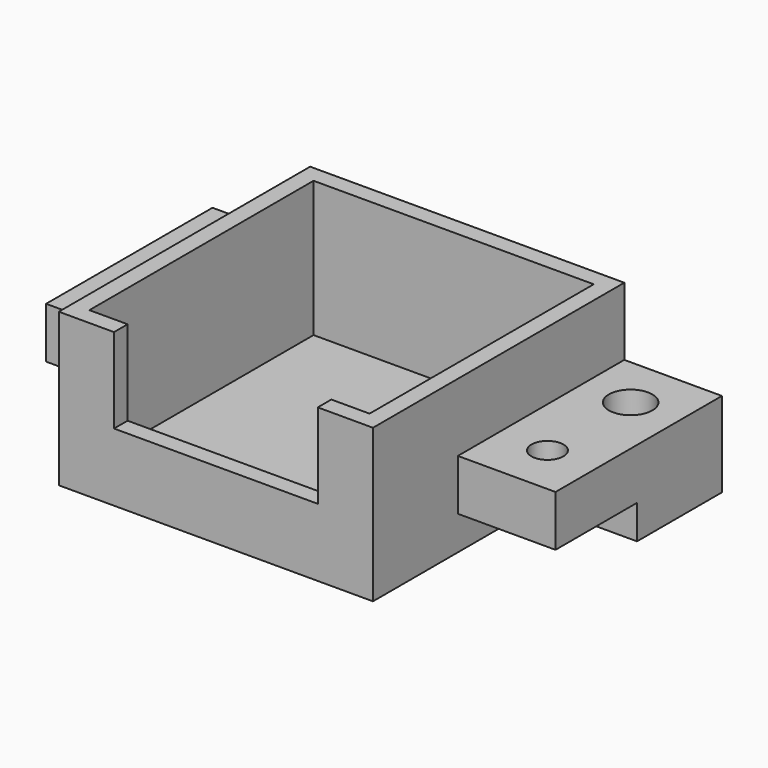
from build123d import *

# Parameters (mm, degrees)
F0_W      = 29.36875
F0_H      = 29.36875
F0_W_2    = 26.19375
F0_H_2    = 26.19375
F1_DEPTH  = 14.2875
F2_W      = 26.19375
F2_H      = 26.19375
F3_DEPTH  = 1.5875
F7_W      = 19.05
F7_H      = 7.9375
F8_DEPTH  = 1.5875
F9_R      = 1.5
F10_DEPTH = 4.7625
F11_R     = 2.032
F12_DEPTH = 7.9375


with BuildPart() as f1:
    # F0 (on Top) → F1 (new body)
    with BuildSketch(Plane.XY):
        Rectangle(F0_W, F0_H)
        Rectangle(F0_W_2, F0_H_2, mode=Mode.SUBTRACT)
    extrude(amount=F1_DEPTH)

    # F2 (on face) → F3 (join)
    with BuildSketch(Plane(origin=(0, 0, 0), x_dir=(1, 0, 0), z_dir=(0, 0, -1))):
        Rectangle(F2_W, F2_H)
    extrude(amount=-F3_DEPTH)

    # F4: union 

    # F7 (on face) → F8 (cut, through all)
    with BuildSketch(Plane.XZ.offset(14.684375)):
        with Locations((0, 10.31875)):
            Rectangle(F7_W, F7_H)
    extrude(amount=-F8_DEPTH, mode=Mode.SUBTRACT)

    # F9 (on face) → F10 (join)
    with BuildSketch(Plane(origin=(0, 0, 3.175), x_dir=(1, 0, 0), z_dir=(0, 0, -1))):
        Polygon((23.8125, 4.7625), (19.2484375, 4.7625), (14.684375, 4.7625), (14.684375, -4.7625), (19.2484375, -4.7625), (23.8125, -4.7625), align=None)
        with Locations((19.2484375, 0)):
            Circle(F9_R, mode=Mode.SUBTRACT)
        Polygon((-19.2484375, -4.7625), (-14.684375, -4.7625), (-14.684375, 4.7625), (-19.2484375, 4.7625), (-23.8125, 4.7625), (-23.8125, -4.7625), align=None)
        with Locations((-19.2484375, 0)):
            Circle(F9_R, mode=Mode.SUBTRACT)
    extrude(amount=-F10_DEPTH)

    # F11 (on face) → F12 (join, through all)
    with BuildSketch(Plane(origin=(0, 0, 0), x_dir=(1, 0, 0), z_dir=(0, 0, -1))):
        Polygon((-23.8125, -14.684375), (-19.2484375, -14.684375), (-14.684375, -14.684375), (-14.684375, -4.7625), (-19.2484375, -4.7625), (-23.8125, -4.7625), align=None)
        with Locations((-19.2484375, -9.7234375)):
            Circle(F11_R, mode=Mode.SUBTRACT)
        Polygon((14.684375, -14.684375), (19.2484375, -14.684375), (23.8125, -14.684375), (23.8125, -4.7625), (19.2484375, -4.7625), (14.684375, -4.7625), align=None)
        with Locations((19.2484375, -9.7234375)):
            Circle(F11_R, mode=Mode.SUBTRACT)
    extrude(amount=-F12_DEPTH)


solid = f1.part
